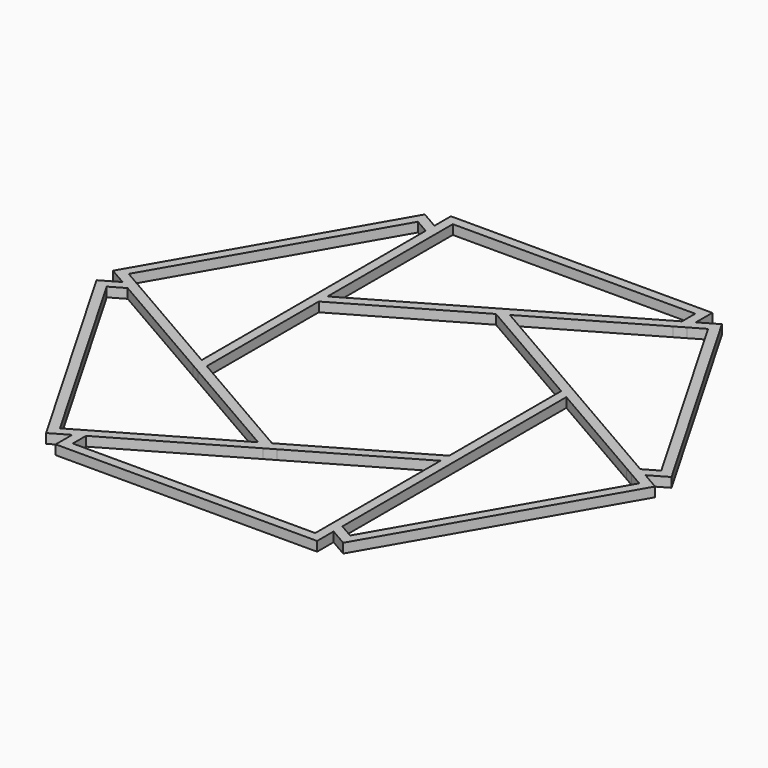
from build123d import *

# Parameters (mm, degrees)
F1_DEPTH = 2


# Not quite as in the source:
# - a feature names something its author has since deleted; it is built from what else it names


with BuildPart() as f1:
    # F0 (on Top) → F1 (new body)
    with BuildSketch(Plane.XY):
        Polygon((27.5, 51.9615242271), (-27.5, 51.9615242271), (-27.5, 47.6313972081), (-25.5, 46.4766966698), (-25.5, 49.9615242271), (25.5, 49.9615242271), (25.5, 46.4766966698), (27.5, 47.6313972081), align=None)
        Polygon((-25.5, 46.4766966698), (-27.5, 47.6313972081), (-27.5, 45.3219961314), (-25.5, 44.167295593), align=None)
        Polygon((-27.5, 45.3219961314), (-27.5, 47.6313972081), (-31.25, 49.7964607176), (-58.75, 2.1650635095), (-55, 0), (-53, 1.1547005384), (-56.0179491924, 2.897114317), (-30.5179491924, 47.06440991), align=None)
        Polygon((31.25, 49.7964607176), (27.5, 47.6313972081), (27.5, 45.3219961314), (30.5179491924, 47.06440991), (56.0179491924, 2.897114317), (53, 1.1547005384), (55, 0), (58.75, 2.1650635095), align=None)
        Polygon((27.5, 45.3219961314), (27.5, 47.6313972081), (25.5, 46.4766966698), (25.5, 44.167295593), align=None)
        Polygon((-25.5, 44.167295593), (-27.5, 45.3219961314), (-27.5, 15.8771324027), (-25.5, 17.0318329411), align=None)
        Polygon((25.5, 44.167295593), (25.5, 46.4766966698), (0, 31.7542648054), (2, 30.5995642671), align=None)
        Polygon((-25.5, 17.0318329411), (-27.5, 15.8771324027), (-27.5, 13.567731326), (-25.5, 14.7224318643), align=None)
        Polygon((2, 30.5995642671), (0, 31.7542648054), (-2, 30.5995642671), (0, 29.4448637287), align=None)
        Polygon((-25.5, 14.7224318643), (-27.5, 13.567731326), (-27.5, -13.567731326), (-25.5, -14.7224318643), align=None)
        Polygon((-2, 30.5995642671), (-25.5, 17.0318329411), (-25.5, 14.7224318643), (0, 29.4448637287), align=None)
        Polygon((-53, -1.1547005384), (-55, 0), (-58.75, -2.1650635095), (-31.25, -49.7964607176), (-27.5, -47.6313972081), (-27.5, -45.3219961314), (-30.5179491924, -47.06440991), (-56.0179491924, -2.897114317), align=None)
        Polygon((-53, 1.1547005384), (-55, 0), (-53, -1.1547005384), (-51, 0), align=None)
        Polygon((25.5, 17.0318329411), (2, 30.5995642671), (0, 29.4448637287), (25.5, 14.7224318643), align=None)
        Polygon((53, -1.1547005384), (55, 0), (53, 1.1547005384), (51, 0), align=None)
        Polygon((58.75, -2.1650635095), (55, 0), (53, -1.1547005384), (56.0179491924, -2.897114317), (30.5179491924, -47.06440991), (27.5, -45.3219961314), (27.5, -47.6313972081), (31.25, -49.7964607176), align=None)
        Polygon((-25.5, -14.7224318643), (-27.5, -13.567731326), (-27.5, -15.8771324027), (-25.5, -17.0318329411), align=None)
        Polygon((-27.5, -15.8771324027), (-27.5, -13.567731326), (-51, 0), (-53, -1.1547005384), align=None)
        Polygon((27.5, 15.8771324027), (25.5, 17.0318329411), (25.5, 14.7224318643), (27.5, 13.567731326), align=None)
        Polygon((51, 0), (53, 1.1547005384), (27.5, 15.8771324027), (27.5, 13.567731326), align=None)
        Polygon((0, -29.4448637287), (-25.5, -14.7224318643), (-25.5, -17.0318329411), (-2, -30.5995642671), align=None)
        Polygon((27.5, 13.567731326), (25.5, 14.7224318643), (25.5, -14.7224318643), (27.5, -13.567731326), align=None)
        Polygon((2, -30.5995642671), (0, -29.4448637287), (-2, -30.5995642671), (0, -31.7542648054), align=None)
        Polygon((25.5, -14.7224318643), (0, -29.4448637287), (2, -30.5995642671), (25.5, -17.0318329411), align=None)
        Polygon((-27.5, -45.3219961314), (-27.5, -47.6313972081), (-25.5, -46.4766966698), (-25.5, -44.167295593), align=None)
        Polygon((-25.5, -46.4766966698), (-27.5, -47.6313972081), (-27.5, -51.9615242271), (27.5, -51.9615242271), (27.5, -47.6313972081), (25.5, -46.4766966698), (25.5, -49.9615242271), (-25.5, -49.9615242271), align=None)
        Polygon((27.5, -13.567731326), (25.5, -14.7224318643), (25.5, -17.0318329411), (27.5, -15.8771324027), align=None)
        Polygon((25.5, -46.4766966698), (27.5, -47.6313972081), (27.5, -45.3219961314), (25.5, -44.167295593), align=None)
        Polygon((0, -31.7542648054), (-2, -30.5995642671), (-25.5, -44.167295593), (-25.5, -46.4766966698), align=None)
        Polygon((27.5, -15.8771324027), (25.5, -17.0318329411), (25.5, -44.167295593), (27.5, -45.3219961314), align=None)
    extrude(amount=F1_DEPTH)


solid = f1.part
